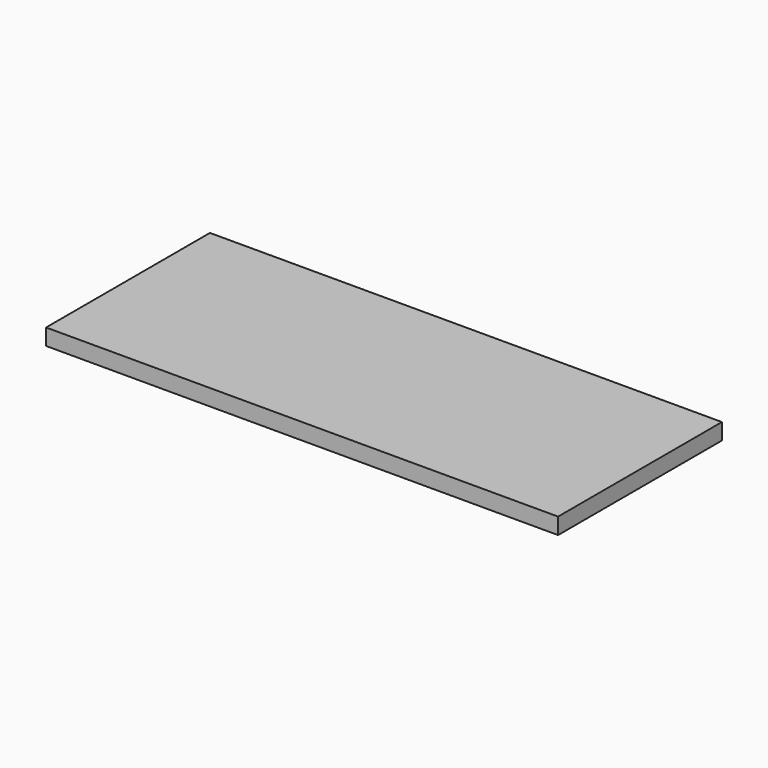
from build123d import *

# Parameters (mm, degrees)
F0_W     = 698.5
F0_H     = 279.4
F1_DEPTH = 22.225


# Not quite as in the source:
# - a length typed as a fraction of an inch, garbled in the dataset ("3 / 203.2 mm" for 3/8 in), is restored


with BuildPart() as f1:
    # F0 (on Top) → F1 (new body)
    with BuildSketch(Plane.XY):
        with Locations((349.25, 139.7)):
            Rectangle(F0_W, F0_H)
    extrude(amount=F1_DEPTH)


solid = f1.part
